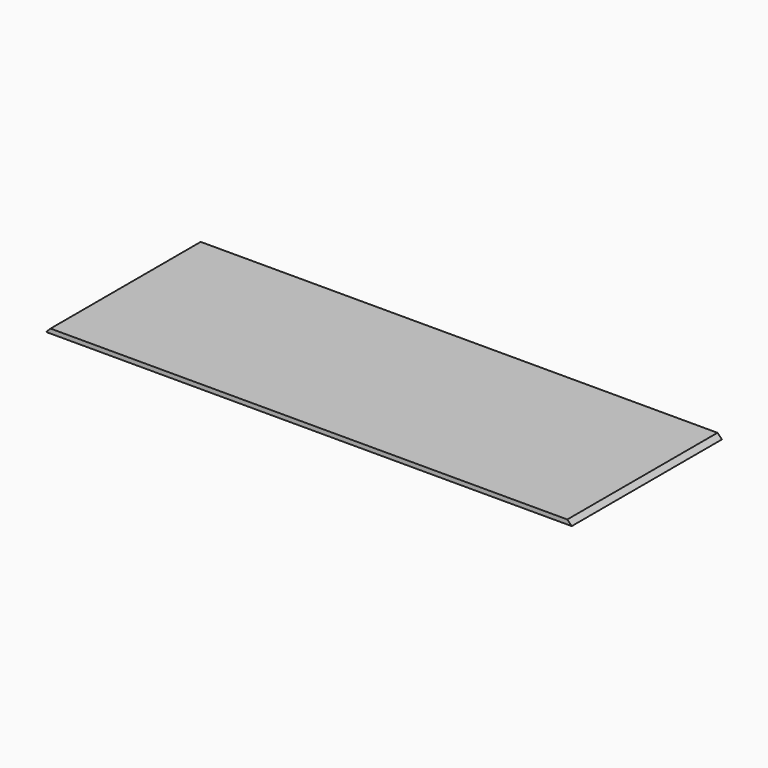
from build123d import *

# Parameters (mm, degrees)
F0_W     = 2133.6
F0_H     = 762
F1_DEPTH = 17.99844
F2_SIZE  = 17.99843


# Not quite as in the source:
# - a fillet or chamfer is up to 0.001 mm smaller than in the source, because OpenCascade refuses the exact size


with BuildPart() as f1:
    # F0 (on Top) → F1 (new body)
    with BuildSketch(Plane.XY):
        with Locations((1066.8, 381)):
            Rectangle(F0_W, F0_H)
    extrude(amount=F1_DEPTH)

    # F2 (size 17.99844 in the source; OpenCascade refuses exactly that, so slightly less here)
    f2_edges = [f1.edges().sort_by_distance(p)[0] for p in [
        (2133.6, 381, 17.99844),
        (0, 381, 17.99844),
    ]]
    chamfer(f2_edges, length=F2_SIZE)


solid = f1.part
